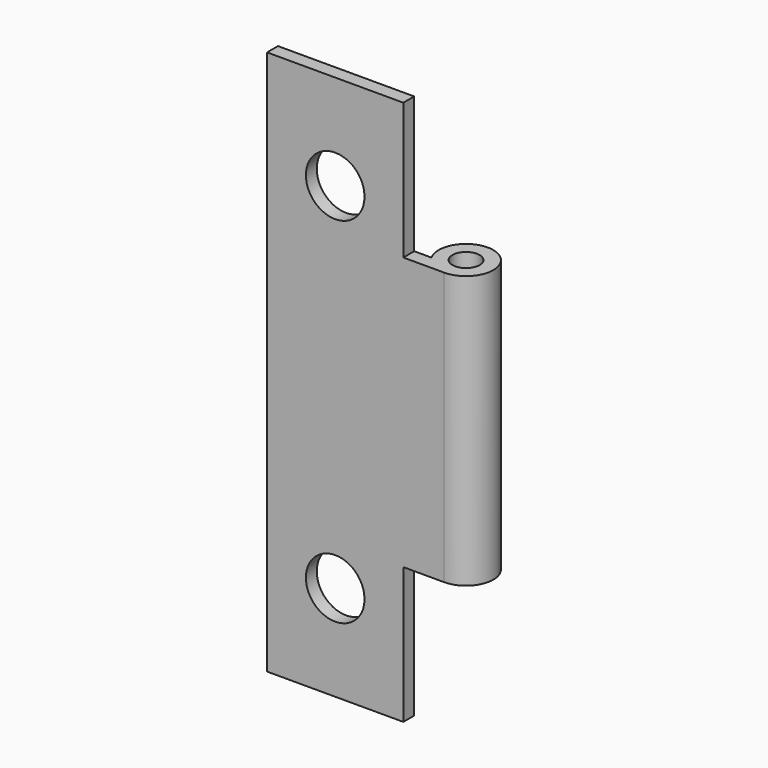
from build123d import *

# Parameters (mm, degrees)
F0_W     = 3
F0_H     = 20
F1_DEPTH = 1
F2_W     = 1
F2_H     = 20
F5_D     = 4.3
F5_DEPTH = 2.5
F5_TIP   = 1.2918503309


# Not quite as in the source:
# - a feature names something its author has since deleted; it is built from what else it names


with BuildPart() as f1:
    # F0 (on Front) → F1 (new body)
    with BuildSketch(Plane.XZ):
        Polygon((5, 10), (5, 20), (-5, 20), (-5, -20), (5, -20), (5, -10), align=None)
        with Locations((6.5, 0)):
            Rectangle(F0_W, F0_H)
    extrude(amount=F1_DEPTH)

    # F2 (on face) → F3 (revolve)
    with BuildSketch(Plane.YZ.offset(8)):
        with Locations((-0.5, 0)):
            Rectangle(F2_W, F2_H)
    revolve(axis=Axis((8, 1, 0), (0, 0, 1)))

    # F5
    with Locations(Plane.XZ.offset(1)):
        with Locations((0, 13), (0, -13)):
            Hole(F5_D / 2, depth=F5_DEPTH)
            with Locations((0, 0, -(F5_DEPTH + F5_TIP / 2))):  # 118° drill point
                Cone(0, F5_D / 2, F5_TIP, mode=Mode.SUBTRACT)


solid = f1.part
